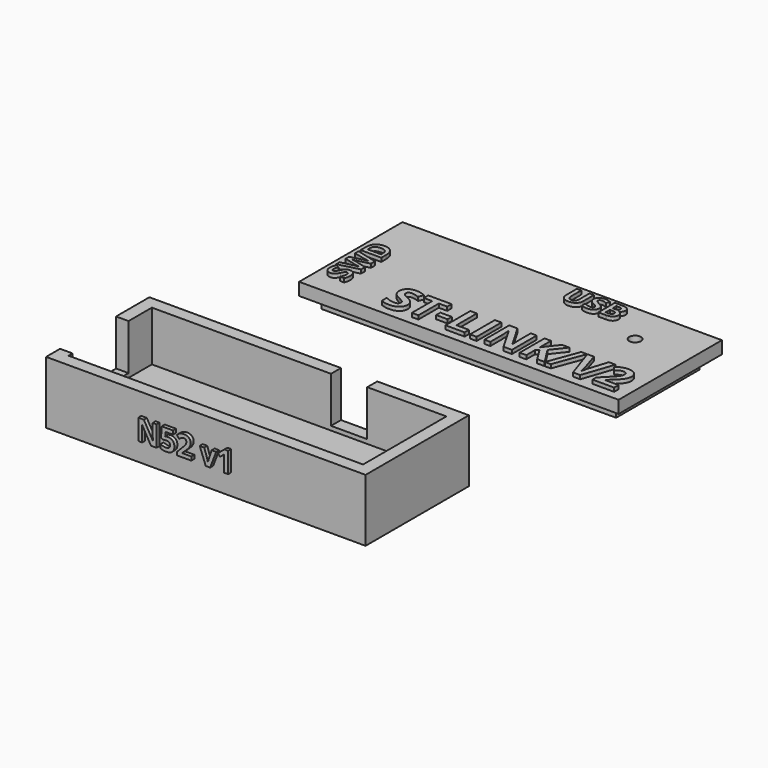
from build123d import *

# Parameters (mm, degrees)
F1_DEPTH       = 3
F2_DEPTH       = 15
F0_W           = 8.7
F0_H           = 3
F0_W_2         = 3
F0_H_2         = 16.8
F3_DEPTH       = 4
F0_W_3         = 76.7
F0_H_3         = 31
F0_W_4         = 70.7
F0_H_4         = 25
F4_DEPTH       = 3
F0_W_5         = 62.7
F0_H_5         = 17
F5_DEPTH       = 6
F6_SIZE        = 2.99999
F7_R           = 1.4
F7_TEXT_SIZE   = 10.4166666667
F7_TEXT_SIZE_2 = 6.9444444444
F8_DEPTH       = 0.9
F9_DEPTH       = 6.901
F10_TEXT_SIZE  = 6.9444444444
F11_DEPTH      = 0.9
F12_TEXT_SIZE  = 6.9444444444
F13_DEPTH      = 0.9


# Not quite as in the source:
# - a fillet or chamfer is up to 0.001 mm smaller than in the source, because OpenCascade refuses the exact size
# - Text() gives the source's letters only with a copy of the font that has no kerning and outlines rounded to 1/6400 em; it was checked with that copy


with BuildPart() as f1:
    # F0 (on Top) → F1 (new body)
    with BuildSketch(Plane.XY):
        Polygon((-30.5477925837, -11.0107796669), (-30.5477925837, -12.2107796669), (40.1522074163, -12.2107796669), (40.1522074163, 12.7892203331), (21.1522074163, 12.7892203331), (12.4522074163, 12.7892203331), (-30.5477925837, 12.7892203331), (-30.5477925837, 5.7892203331), align=None)
    extrude(amount=F1_DEPTH)

    # F0 (on Top) → F2 (join)
    with BuildSketch(Plane.XY):
        Polygon((-33.5477925837, 5.7892203331), (-30.5477925837, 5.7892203331), (-30.5477925837, 12.7892203331), (12.4522074163, 12.7892203331), (12.4522074163, 15.7892203331), (-33.5477925837, 15.7892203331), align=None)
        Polygon((40.1522074163, -12.2107796669), (-30.5477925837, -12.2107796669), (-30.5477925837, -11.0107796669), (-33.5477925837, -11.0107796669), (-33.5477925837, -15.2107796669), (43.1522074163, -15.2107796669), (43.1522074163, 15.7892203331), (21.1522074163, 15.7892203331), (21.1522074163, 12.7892203331), (40.1522074163, 12.7892203331), align=None)
    extrude(amount=F2_DEPTH)

    # F0 (on Top) → F3 (join)
    with BuildSketch(Plane.XY):
        with Locations((16.8022074163, 14.2892203331)):
            Rectangle(F0_W, F0_H)
        with Locations((-32.0477925837, -2.6107796669)):
            Rectangle(F0_W_2, F0_H_2)
    extrude(amount=F3_DEPTH)

    # F12 (on face) → F13 (join)
    with BuildSketch(Plane.XZ.offset(15.2107796669)):
        with Locations((-11.3237847222, 5)):
            Text('N52 v1', F12_TEXT_SIZE, font='Open Sans', font_style=FontStyle.BOLD, text_align=(TextAlign.LEFT, TextAlign.BOTTOM))
    extrude(amount=F13_DEPTH)


with BuildPart() as f4:
    # F0 (on Top) → F4 (new body)
    with BuildSketch(Plane.XY):
        with Locations((4.8022074163, 76.2180483513)):
            Rectangle(F0_W_3, F0_H_3)
        with Locations((4.8022074163, 76.2180483513)):
            Rectangle(F0_W_4, F0_H_4, mode=Mode.SUBTRACT)
    extrude(amount=-F4_DEPTH)



with BuildPart() as f4b:
    # F0 (on Top) → F4, piece 2 (new body)
    with BuildSketch(Plane.XY):
        with Locations((4.8022074163, 76.2180483513)):
            Rectangle(F0_W_5, F0_H_5)
    extrude(amount=-F4_DEPTH)


with BuildPart() as f4_1:
    add(f4.part)

    add(f4b.part)  # F5 merges F4b
    # F0 (on Top) → F5 (join)
    with BuildSketch(Plane.XY):
        with Locations((4.8022074163, 76.2180483513)):
            Rectangle(F0_W_4, F0_H_4)
        with Locations((4.8022074163, 76.2180483513)):
            Rectangle(F0_W_5, F0_H_5, mode=Mode.SUBTRACT)
    extrude(amount=-F5_DEPTH)

    # F6 (size 3 in the source; OpenCascade refuses exactly that, so slightly less here)
    f6_edges = [f4_1.edges().sort_by_distance(p)[0] for p in [
        (-26.547793, 76.218048, -6),
        (4.802207, 84.718048, -6),
        (4.802207, 67.718048, -6),
        (36.152207, 76.218048, -6),
    ]]
    chamfer(f6_edges, length=F6_SIZE)

    # F7 (on face) → F8 (join)
    with BuildSketch(Plane.XY):
        with Locations((30.1522074163, 81.9180483513)):
            Circle(F7_R)
        with Locations((-16.0515686254, 62.7180483513)):
            Text('ST-LINK/V2', F7_TEXT_SIZE, font='Open Sans', font_style=FontStyle.BOLD, text_align=(TextAlign.LEFT, TextAlign.BOTTOM))
        with Locations((9.3826235859, 84.7180483513)):
            Text('USB', F7_TEXT_SIZE_2, font='Open Sans', font_style=FontStyle.BOLD, text_align=(TextAlign.LEFT, TextAlign.BOTTOM))
        with Locations(Location((-26.5477925837, 65.4545500875), (0, 0, 90))):
            Text('SWD', F7_TEXT_SIZE_2, font='Open Sans', font_style=FontStyle.BOLD, text_align=(TextAlign.LEFT, TextAlign.BOTTOM))
    extrude(amount=F8_DEPTH)

    # F9 (cut, through all): a face of the model
    f9_faces = [f4_1.faces().sort_by_distance(p)[0] for p in [
        (30.1522074163, 81.9180483513, 0.9),
    ]]
    extrude(f9_faces, amount=-F9_DEPTH, mode=Mode.SUBTRACT)

    # F10 (on face) → F11 (join)
    with BuildSketch(Plane(origin=(0, 0, -3), x_dir=(1, 0, 0), z_dir=(0, 0, -1))):
        with Locations((-6.5215773059, -78.7180483513)):
            Text('N52 v1', F10_TEXT_SIZE, font='Open Sans', font_style=FontStyle.BOLD, text_align=(TextAlign.LEFT, TextAlign.BOTTOM))
    extrude(amount=F11_DEPTH)


solid = Compound([f1.part, f4_1.part])
